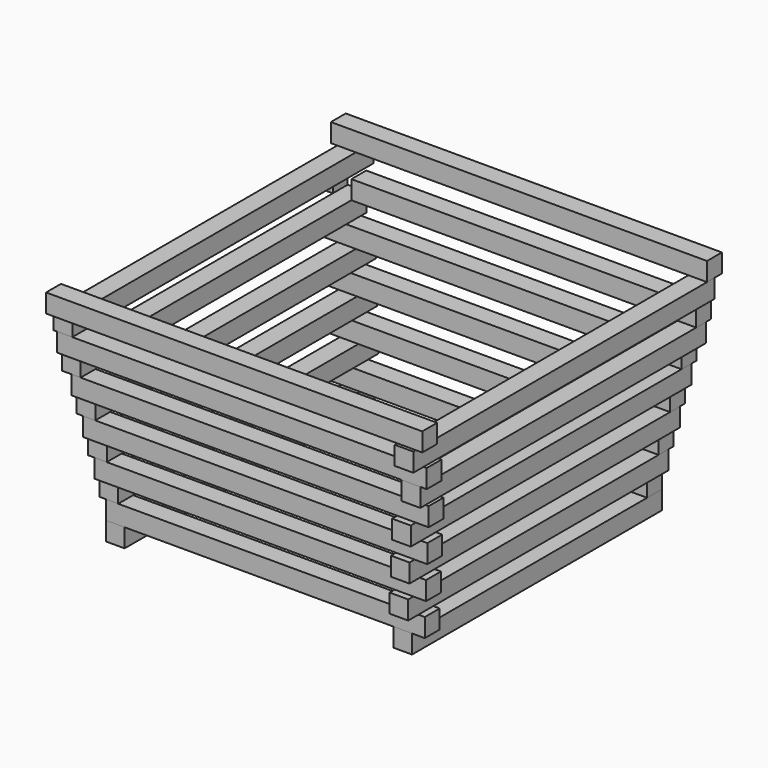
from build123d import *

# Parameters (mm, degrees)
F1_DEPTH  = 3.7041666667
F2_W      = 2.54
F2_H      = 3.7041666667
F2_W_2    = 3.7041666667
F3_DEPTH  = 3.7041666667
F4_W      = 3.7041666667
F4_H      = 2.54
F4_H_2    = 3.7041666667
F5_DEPTH  = 3.7041666667
F4_W_2    = 2.4341666667
F6_W      = 3.7041666667
F6_H      = 2.4341666667
F7_DEPTH  = 3.7041666667
F6_H_2    = 3.7041666667
F6_W_2    = 2.54
F8_W      = 3.7041666667
F8_H      = 2.54
F8_H_2    = 3.7041666667
F9_DEPTH  = 3.7041666667
F8_W_2    = 2.4341666667
F10_W     = 3.7041666667
F10_H     = 3.7041666667
F10_W_2   = 2.54
F11_DEPTH = 3.7041666667
F10_H_2   = 2.4341666667
F12_W     = 3.7041666667
F12_H     = 3.7041666667
F12_H_2   = 2.54
F13_DEPTH = 3.7041666667
F12_W_2   = 2.4341666667
F14_W     = 3.7041666667
F14_H     = 3.7041666667
F14_W_2   = 2.54
F15_DEPTH = 3.7041666667
F14_H_2   = 2.4341666667
F16_W     = 3.7041666667
F16_H     = 3.7041666667
F16_H_2   = 1.27
F17_DEPTH = 3.7041666667
F16_W_2   = 1.7991666667
F18_W     = 1.27
F18_H     = 3.7041666667
F19_DEPTH = 3.7041666667
F18_W_2   = 3.7041666667
F18_H_2   = 2.4341666667
F21_DEPTH = 3.7041666667
F20_W     = 3.0691666667
F20_H     = 3.7041666667
F22_W     = 1.27
F22_H     = 3.7041666667
F22_W_2   = 3.7041666667
F23_DEPTH = 3.7041666667
F22_H_2   = 1.7991666667


# Not quite as in the source:
# - a feature names something its author has since deleted; it is built from what else it names


with BuildPart() as f1:
    # F0 (on Top) → F1 (new body)
    with BuildSketch(Plane.XY):
        Polygon((30.48, 31.115), (26.7758333333, 31.115), (26.7758333333, -6.985), (26.7758333333, -31.115), (30.48, -31.115), align=None)
    extrude(amount=F1_DEPTH)


with BuildPart() as f1b:
    # F0 (on Top) → F1, piece 2 (new body)
    with BuildSketch(Plane.XY):
        Polygon((-26.7758333333, -31.115), (-26.7758333333, 6.985), (-26.7758333333, 31.115), (-30.48, 31.115), (-30.48, -31.115), align=None)
    extrude(amount=F1_DEPTH)


with BuildPart() as f3:
    # F2 (on face) → F3 (new body)
    with BuildSketch(Plane.XY.offset(3.7041666667)):
        Polygon((-26.7758333333, 31.115), (-26.7758333333, 27.4108333333), (0, 27.4108333333), (30.48, 27.4108333333), (30.48, 31.115), align=None)
        with Locations((-31.75, 29.2629166667)):
            Rectangle(F2_W, F2_H)
        with Locations((-28.6279166667, 29.2629166667)):
            Rectangle(F2_W_2, F2_H)
    extrude(amount=F3_DEPTH)


with BuildPart() as f3b:
    # F2 (on face) → F3, piece 2 (new body)
    with BuildSketch(Plane.XY.offset(3.7041666667)):
        with Locations((-28.6279166667, -29.2629166667)):
            Rectangle(F2_W_2, F2_H)
        Polygon((-26.7758333333, -27.4108333333), (-26.7758333333, -31.115), (33.02, -31.115), (33.02, -27.4108333333), (0, -27.4108333333), align=None)
    extrude(amount=F3_DEPTH)


with BuildPart() as f5:
    # F4 (on face) → F5 (new body)
    with BuildSketch(Plane.XY.offset(7.4083333333)):
        Polygon((-28.0458333333, 27.4108333333), (-31.75, 27.4108333333), (-31.75, -31.115), (-28.0458333333, -31.115), (-28.0458333333, 0), align=None)
        with Locations((-29.8979166667, 32.385)):
            Rectangle(F4_W, F4_H)
        with Locations((-29.8979166667, 29.2629166667)):
            Rectangle(F4_W, F4_H_2)
    extrude(amount=F5_DEPTH)


with BuildPart() as f5b:
    # F4 (on face) → F5, piece 2 (new body)
    with BuildSketch(Plane.XY.offset(7.4083333333)):
        with Locations((29.2629166667, 29.2629166667)):
            Rectangle(F4_W_2, F4_H_2)
        Polygon((30.48, 27.4108333333), (28.0458333333, 27.4108333333), (28.0458333333, 0), (28.0458333333, -33.655), (31.75, -33.655), (31.75, 31.115), (30.48, 31.115), align=None)
    extrude(amount=F5_DEPTH)


with BuildPart() as f7:
    # F6 (on face) → F7 (new body)
    with BuildSketch(Plane.XY.offset(11.1125)):
        Polygon((0, -28.6808333333), (-28.0458333333, -28.6808333333), (-28.0458333333, -31.115), (-31.75, -31.115), (-31.75, -32.385), (34.29, -32.385), (34.29, -28.6808333333), align=None)
        with Locations((-29.8979166667, -29.8979166667)):
            Rectangle(F6_W, F6_H)
    extrude(amount=F7_DEPTH)


with BuildPart() as f7b:
    # F6 (on face) → F7, piece 2 (new body)
    with BuildSketch(Plane.XY.offset(11.1125)):
        Polygon((31.75, 32.385), (-28.0458333333, 32.385), (-28.0458333333, 28.6808333333), (0, 28.6808333333), (31.75, 28.6808333333), align=None)
        with Locations((-29.8979166667, 30.5329166667)):
            Rectangle(F6_W, F6_H_2)
        with Locations((-33.02, 30.5329166667)):
            Rectangle(F6_W_2, F6_H_2)
    extrude(amount=F7_DEPTH)


with BuildPart() as f9:
    # F8 (on face) → F9 (new body)
    with BuildSketch(Plane.XY.offset(14.8166666667)):
        Polygon((-29.3158333333, -32.385), (-29.3158333333, 0), (-29.3158333333, 28.6808333333), (-33.02, 28.6808333333), (-33.02, -32.385), align=None)
        with Locations((-31.1679166667, 33.655)):
            Rectangle(F8_W, F8_H)
        with Locations((-31.1679166667, 30.5329166667)):
            Rectangle(F8_W, F8_H_2)
    extrude(amount=F9_DEPTH)


with BuildPart() as f9b:
    # F8 (on face) → F9, piece 2 (new body)
    with BuildSketch(Plane.XY.offset(14.8166666667)):
        with Locations((30.5329166667, 30.5329166667)):
            Rectangle(F8_W_2, F8_H_2)
        Polygon((29.3158333333, -34.925), (33.02, -34.925), (33.02, 32.385), (31.75, 32.385), (31.75, 28.6808333333), (29.3158333333, 28.6808333333), (29.3158333333, 0), align=None)
    extrude(amount=F9_DEPTH)


with BuildPart() as f11:
    # F10 (on face) → F11 (new body)
    with BuildSketch(Plane.XY.offset(18.5208333333)):
        Polygon((-29.3158333333, 29.9508333333), (0, 29.9508333333), (33.02, 29.9508333333), (33.02, 33.655), (-29.3158333333, 33.655), align=None)
        with Locations((-31.1679166667, 31.8029166667)):
            Rectangle(F10_W, F10_H)
        with Locations((-34.29, 31.8029166667)):
            Rectangle(F10_W_2, F10_H)
    extrude(amount=F11_DEPTH)


with BuildPart() as f11b:
    # F10 (on face) → F11, piece 2 (new body)
    with BuildSketch(Plane.XY.offset(18.5208333333)):
        with Locations((-31.1679166667, -31.1679166667)):
            Rectangle(F10_W, F10_H_2)
        Polygon((35.56, -29.9508333333), (0, -29.9508333333), (-29.3158333333, -29.9508333333), (-29.3158333333, -32.385), (-33.02, -32.385), (-33.02, -33.655), (35.56, -33.655), align=None)
    extrude(amount=F11_DEPTH)


with BuildPart() as f13:
    # F12 (on face) → F13 (new body)
    with BuildSketch(Plane.XY.offset(22.225)):
        Polygon((-30.5858333333, -33.655), (-30.5858333333, 0), (-30.5858333333, 29.9508333333), (-34.29, 29.9508333333), (-34.29, -33.655), align=None)
        with Locations((-32.4379166667, 31.8029166667)):
            Rectangle(F12_W, F12_H)
        with Locations((-32.4379166667, 34.925)):
            Rectangle(F12_W, F12_H_2)
    extrude(amount=F13_DEPTH)


with BuildPart() as f13b:
    # F12 (on face) → F13, piece 2 (new body)
    with BuildSketch(Plane.XY.offset(22.225)):
        Polygon((34.29, -36.195), (34.29, 33.655), (33.02, 33.655), (33.02, 29.9508333333), (30.5858333333, 29.9508333333), (30.5858333333, 0), (30.5858333333, -36.195), align=None)
        with Locations((31.8029166667, 31.8029166667)):
            Rectangle(F12_W_2, F12_H)
    extrude(amount=F13_DEPTH)


with BuildPart() as f15:
    # F14 (on face) → F15 (new body)
    with BuildSketch(Plane.XY.offset(25.9291666667)):
        Polygon((34.29, 34.925), (-30.5858333333, 34.925), (-30.5858333333, 31.2208333333), (0, 31.2208333333), (34.29, 31.2208333333), align=None)
        with Locations((-32.4379166667, 33.0729166667)):
            Rectangle(F14_W, F14_H)
        with Locations((-35.56, 33.0729166667)):
            Rectangle(F14_W_2, F14_H)
    extrude(amount=F15_DEPTH)


with BuildPart() as f15b:
    # F14 (on face) → F15, piece 2 (new body)
    with BuildSketch(Plane.XY.offset(25.9291666667)):
        with Locations((-32.4379166667, -32.4379166667)):
            Rectangle(F14_W, F14_H_2)
        Polygon((0, -31.2208333333), (-30.5858333333, -31.2208333333), (-30.5858333333, -33.655), (-34.29, -33.655), (-34.29, -34.925), (36.83, -34.925), (36.83, -31.2208333333), align=None)
    extrude(amount=F15_DEPTH)


with BuildPart() as f17:
    # F16 (on face) → F17 (new body)
    with BuildSketch(Plane.XY.offset(29.6333333333)):
        Polygon((-32.4908333333, -34.925), (-32.4908333333, 0), (-32.4908333333, 31.2208333333), (-36.195, 31.2208333333), (-36.195, -34.925), align=None)
        with Locations((-34.3429166667, 33.0729166667)):
            Rectangle(F16_W, F16_H)
        with Locations((-34.3429166667, 35.56)):
            Rectangle(F16_W, F16_H_2)
    extrude(amount=F17_DEPTH)


with BuildPart() as f17b:
    # F16 (on face) → F17, piece 2 (new body)
    with BuildSketch(Plane.XY.offset(29.6333333333)):
        with Locations((33.3904166667, 33.0729166667)):
            Rectangle(F16_W_2, F16_H)
        Polygon((36.195, -36.195), (36.195, 34.925), (34.29, 34.925), (34.29, 31.2208333333), (32.4908333333, 31.2208333333), (32.4908333333, 0), (32.4908333333, -36.195), align=None)
    extrude(amount=F17_DEPTH)


with BuildPart() as f19:
    # F18 (on face) → F19 (new body)
    with BuildSketch(Plane.XY.offset(33.3375)):
        with Locations((-36.83, 34.3429166667)):
            Rectangle(F18_W, F18_H)
    extrude(amount=F19_DEPTH)


with BuildPart() as f19b:
    # F18 (on face) → F19, piece 2 (new body)
    with BuildSketch(Plane.XY.offset(33.3375)):
        Polygon((36.195, 36.195), (-32.4908333333, 36.195), (-32.4908333333, 32.4908333333), (0, 32.4908333333), (36.195, 32.4908333333), align=None)
    extrude(amount=F19_DEPTH)


with BuildPart() as f19c:
    # F18 (on face) → F19, piece 3 (new body)
    with BuildSketch(Plane.XY.offset(33.3375)):
        with Locations((-34.3429166667, -33.7079166667)):
            Rectangle(F18_W_2, F18_H_2)
        Polygon((0, -32.4908333333), (-32.4908333333, -32.4908333333), (-32.4908333333, -34.925), (-36.195, -34.925), (-36.195, -36.195), (37.465, -36.195), (37.465, -32.4908333333), align=None)
    extrude(amount=F19_DEPTH)


with BuildPart() as f21:
    # F20 (on face) → F21 (new body)
    with BuildSketch(Plane.XY.offset(37.0416666667)):
        Polygon((-33.1258333333, -36.195), (-33.1258333333, 0), (-33.1258333333, 38.735), (-36.83, 38.735), (-36.83, -36.195), align=None)
    extrude(amount=F21_DEPTH)


with BuildPart() as f21b:
    # F20 (on face) → F21, piece 2 (new body)
    with BuildSketch(Plane.XY.offset(37.0416666667)):
        Polygon((36.83, -38.735), (36.83, 36.195), (36.195, 36.195), (36.195, 32.4908333333), (33.1258333333, 32.4908333333), (33.1258333333, 0), (33.1258333333, -38.735), align=None)
        with Locations((34.6604166667, 34.3429166667)):
            Rectangle(F20_W, F20_H)
    extrude(amount=F21_DEPTH)


with BuildPart() as f23:
    # F22 (on face) → F23 (new body)
    with BuildSketch(Plane.XY.offset(40.7458333333)):
        Polygon((-33.1258333333, 34.3958333333), (0, 34.3958333333), (36.83, 34.3958333333), (36.83, 38.1), (-33.1258333333, 38.1), align=None)
        with Locations((-37.465, 36.2479166667)):
            Rectangle(F22_W, F22_H)
        with Locations((-34.9779166667, 36.2479166667)):
            Rectangle(F22_W_2, F22_H)
    extrude(amount=F23_DEPTH)


with BuildPart() as f23b:
    # F22 (on face) → F23, piece 2 (new body)
    with BuildSketch(Plane.XY.offset(40.7458333333)):
        with Locations((-34.9779166667, -35.2954166667)):
            Rectangle(F22_W_2, F22_H_2)
        Polygon((38.1, -34.3958333333), (0, -34.3958333333), (-33.1258333333, -34.3958333333), (-33.1258333333, -36.195), (-36.83, -36.195), (-36.83, -38.1), (38.1, -38.1), align=None)
    extrude(amount=F23_DEPTH)


solid = Compound([f1.part, f1b.part, f3.part, f3b.part, f5.part, f5b.part, f7.part, f7b.part, f9.part, f9b.part, f11.part, f11b.part, f13.part, f13b.part, f15.part, f15b.part, f17.part, f17b.part, f19.part, f19b.part, f19c.part, f21.part, f21b.part, f23.part, f23b.part])
